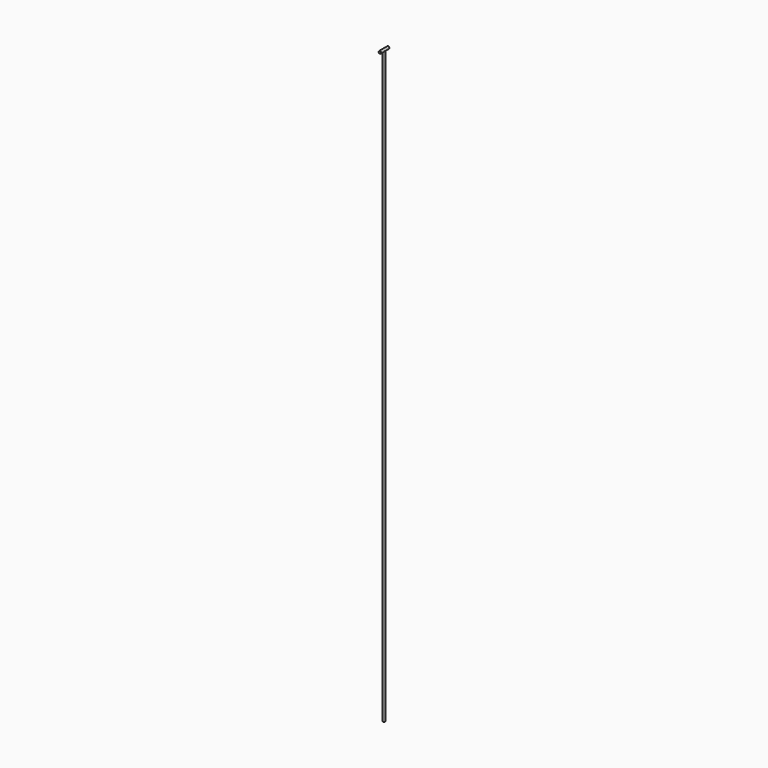
from build123d import *

# Parameters (mm, degrees)
F0_W         = 6.35
F0_H         = 6.35
F0_H_2       = 1466.85
F1_DEPTH     = 3.175
F2_R         = 3.175
F3_DEPTH     = 12.7
F4_T3_DEPTH  = 1489.075
F4_S4_R      = 3.175
F4_T5_DEPTH  = 746
F4_T8_DEPTH  = 1489.075
F4_S9_R      = 3.175
F4_T10_DEPTH = 746
F4_T13_DEPTH = 1489.075
F4_S14_R     = 3.175
F4_T15_DEPTH = 746
F4_T18_DEPTH = 1489.075
F4_S19_R     = 3.175
F4_T20_DEPTH = 746


# Not quite as in the source:
# - a fillet or chamfer that OpenCascade refuses, or shapes differently, is made with other operations: its cross-section is extruded or revolved along the edge and cut away or added


with BuildPart() as f1:
    # F0 (on Front) → F1 (new body, symmetric)
    with BuildSketch(Plane.XZ):
        with Locations((0, 733.425)):
            Rectangle(F0_W, F0_H)
        with Locations((0, -3.175)):
            Rectangle(F0_W, F0_H_2)
    extrude(amount=F1_DEPTH, both=True)

    # F2 (on Front) → F3 (join, symmetric)
    with BuildSketch(Plane.XZ):
        with Locations((0, 736.6)):
            Circle(F2_R)
    extrude(amount=F3_DEPTH, both=True)

    # F4: fillet of radius 3.175 on 4 edges, made by hand


with BuildPart() as f4_tool1:
    # F4_s2 → F4_t3 (new body)
    with BuildSketch(Plane.XY.offset(-744.5375)):
        with BuildLine():
            ThreePointArc((0, -3.175), (2.2450640303, -2.2450640303), (3.175, 0))
            Line((3.175, 0), (3.175, -3.175))
            Line((3.175, -3.175), (0, -3.175))
        make_face()
    extrude(amount=F4_T3_DEPTH)

    # F4_s4 → F4_t5 (cut, symmetric)
    with BuildSketch(Plane.XZ.offset(1.6)):
        with Locations((0, 736.6)):
            Circle(F4_S4_R)
    extrude(amount=F4_T5_DEPTH, both=True, mode=Mode.SUBTRACT)


with BuildPart() as f4_tool6:
    # F4_s7 → F4_t8 (new body)
    with BuildSketch(Plane.XY.offset(-744.5375)):
        with BuildLine():
            ThreePointArc((0, 3.175), (2.2450640303, 2.2450640303), (3.175, 0))
            Line((3.175, 0), (3.175, 3.175))
            Line((3.175, 3.175), (0, 3.175))
        make_face()
    extrude(amount=F4_T8_DEPTH)

    # F4_s9 → F4_t10 (cut, symmetric)
    with BuildSketch(Plane.XZ.offset(-1.6)):
        with Locations((0, 736.6)):
            Circle(F4_S9_R)
    extrude(amount=F4_T10_DEPTH, both=True, mode=Mode.SUBTRACT)


with BuildPart() as f4_tool11:
    # F4_s12 → F4_t13 (new body)
    with BuildSketch(Plane.XY.offset(744.5375)):
        with BuildLine():
            ThreePointArc((-3.175, 0), (-2.2450640303, 2.2450640303), (0, 3.175))
            Line((0, 3.175), (-3.175, 3.175))
            Line((-3.175, 3.175), (-3.175, 0))
        make_face()
    extrude(amount=-F4_T13_DEPTH)

    # F4_s14 → F4_t15 (cut, symmetric)
    with BuildSketch(Plane.XZ.offset(-1.6)):
        with Locations((0, 736.6)):
            Circle(F4_S14_R)
    extrude(amount=F4_T15_DEPTH, both=True, mode=Mode.SUBTRACT)


with BuildPart() as f4_tool16:
    # F4_s17 → F4_t18 (new body)
    with BuildSketch(Plane.XY.offset(744.5375)):
        with BuildLine():
            ThreePointArc((-3.175, 0), (-2.2450640303, -2.2450640303), (0, -3.175))
            Line((0, -3.175), (-3.175, -3.175))
            Line((-3.175, -3.175), (-3.175, 0))
        make_face()
    extrude(amount=-F4_T18_DEPTH)

    # F4_s19 → F4_t20 (cut, symmetric)
    with BuildSketch(Plane.XZ.offset(1.6)):
        with Locations((0, 736.6)):
            Circle(F4_S19_R)
    extrude(amount=F4_T20_DEPTH, both=True, mode=Mode.SUBTRACT)


with BuildPart() as f1_1:
    add(f1.part)

    # F4_t21: cut F4_tool1, F4_tool6, F4_tool11, F4_tool16
    add([f4_tool1.part, f4_tool6.part, f4_tool11.part, f4_tool16.part], mode=Mode.SUBTRACT)


solid = f1_1.part
